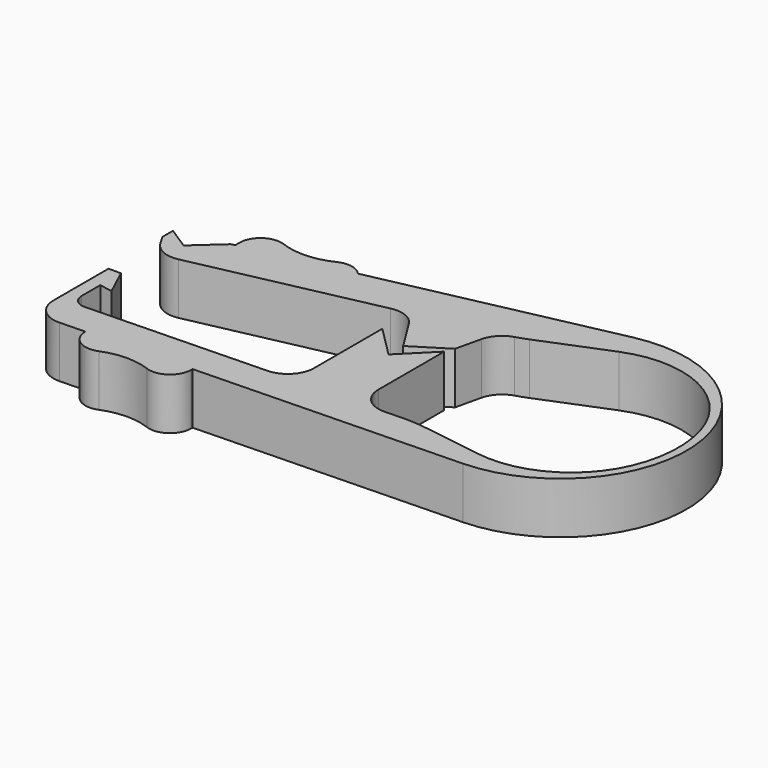
from build123d import *

# Parameters (mm, degrees)
F1_DEPTH     = 5
F2_R         = 12.7
F3_T1_DEPTH  = 5
F3_T3_DEPTH  = 5
F3_T5_DEPTH  = 5
F3_T7_DEPTH  = 5
F3_T9_DEPTH  = 14.2270901057
F3_T11_DEPTH = 18.0454684025
F4_R         = 1.27
F5_R         = 9.652
F6_T1_DEPTH  = 24.5237287856
F6_T3_DEPTH  = 20.8349691576
F6_T5_DEPTH  = 25.4326352389


# Not quite as in the source:
# - a fillet or chamfer that OpenCascade refuses, or shapes differently, is made with other operations: its cross-section is extruded or revolved along the edge and cut away or added


with BuildPart() as f1:
    # F0 (on Top) → F1 (new body)
    with BuildSketch(Plane.XY):
        Polygon((3.3509032068, 2.0938767152), (4.2717468935, 6.0824889279), (5.2645709983, 10.3828825854), (-0.7663700033, 9.1009665025), (-1.7591941081, 4.800572845), (-2.0938767152, 3.3509032068), (0, 0), align=None)
        with BuildLine():
            ThreePointArc((19.0271173058, -10.7843702882), (13.5579507926, -11.3055566189), (8.4773948837, -9.2147746604))
            Line((8.4773948837, -9.2147746604), (3, -9.3617991862))
            Line((3, -9.3617991862), (-3, -9.5228515064))
            Line((-3, -9.5228515064), (-24.13, -10.0900240941))
            Line((-24.13, -10.0900240941), (-24.13, -6.5340240941))
            Line((-24.13, -6.5340240941), (-24.13, -4.0344355705))
            Line((-24.13, -4.0344355705), (-25.33, -4.0344355705))
            Line((-25.33, -4.0344355705), (-25.33, -13.3233871439))
            Line((-25.33, -13.3233871439), (-20.25, -13.1870295128))
            Line((-20.25, -13.1870295128), (-10.09, -12.9143142505))
            Line((-10.09, -12.9143142505), (15.568160115, -12.2255965474))
            ThreePointArc((15.568160115, -12.2255965474), (27.3847553183, 1.4414639293), (12.6972400213, 11.962745157))
            Line((12.6972400213, 11.962745157), (5.2645709983, 10.3828825854))
            Line((5.2645709983, 10.3828825854), (4.2717468935, 6.0824889279))
            Line((4.2717468935, 6.0824889279), (5.7705051289, 6.4010598252))
            ThreePointArc((5.7705051289, 6.4010598252), (10.9582466373, 10.5977114577), (17.6052347625, 11.1826009729))
            ThreePointArc((17.6052347625, 11.1826009729), (26.6461306142, 0.7382983213), (19.0271173058, -10.7843702882))
        make_face()
        Polygon((-24.13, -4.0344355705), (-24.13, -6.5340240941), (-22.86, -6.7579593596), align=None)
        Polygon((-3, -9.5228515064), (3, -9.3617991862), (3, 1.222), (0, -1.778), (-3, 1.222), align=None)
        Polygon((-1.7591941081, 4.800572845), (-0.7663700033, 9.1009665025), (-10.09, 7.1191677681), (-20.25, 4.9595931015), (-20.6003244103, 4.8851293494), (-23.2697767574, 2.48154366), (-25.4, 3.8649268089), (-25.4, 2.5949268089), (-23.9501636865, 0.0837366513), align=None)
        with BuildLine():
            Line((5.7705051289, 6.4010598252), (17.6052347625, 11.1826009729))
            ThreePointArc((17.6052347625, 11.1826009729), (10.9582466373, 10.5977114577), (5.7705051289, 6.4010598252))
        make_face()
        with BuildLine():
            Line((19.0271173058, -10.7843702882), (8.4773948837, -9.2147746604))
            ThreePointArc((8.4773948837, -9.2147746604), (13.5579507926, -11.3055566189), (19.0271173058, -10.7843702882))
        make_face()
        with BuildLine():
            Line((-20.25, 4.9595931015), (-10.09, 7.1191677681))
            Line((-10.09, 7.1191677681), (-10.09, 9.660082633))
            ThreePointArc((-10.09, 9.660082633), (-15.1017802383, 6.9821995552), (-20.25, 9.3873673708))
            Line((-20.25, 9.3873673708), (-20.25, 4.9595931015))
        make_face()
        with BuildLine():
            Line((-10.09, -17.0008412983), (-10.09, -12.9143142505))
            Line((-10.09, -12.9143142505), (-20.25, -13.1870295128))
            Line((-20.25, -13.1870295128), (-20.25, -17.2735565605))
            ThreePointArc((-20.25, -17.2735565605), (-15.2382197617, -14.5956734827), (-10.09, -17.0008412983))
        make_face()
    extrude(amount=F1_DEPTH)

    # F2
    f2_edges = [f1.edges().sort_by_distance(p)[0] for p in [
        (5.770505, 6.40106, 2.5),
        (8.477395, -9.214775, 2.5),
    ]]
    fillet(f2_edges, radius=F2_R)

    # F3: fillet of radius 2.54 on 8 edges, made by hand

    # F3_s2 → F3_t1 (join)
    with BuildSketch(Plane.XY):
        with BuildLine():
            ThreePointArc((5.6695141413, 6.421250807), (4.5433342643, 5.7258928643), (3.9198768127, 4.5583721621))
            Line((3.9198768127, 4.5583721621), (3.6723868163, 4.6155097299))
            Line((3.6723868163, 4.6155097299), (4.024256897, 6.1396264957))
            Line((4.024256897, 6.1396264957), (4.218937324, 6.3309384185))
            ThreePointArc((4.218937324, 6.3309384185), (4.6308698651, 6.4184973831), (5.5969878777, 6.6646762393))
            Line((5.5969878777, 6.6646762393), (5.6695141413, 6.421250807))
        make_face()
    extrude(amount=F3_T1_DEPTH)

    # F3_s4 → F3_t3 (join)
    with BuildSketch(Plane.XY):
        with BuildLine():
            ThreePointArc((-2.0938767152, 3.3509032068), (-3.2128527644, 4.1204303422), (-4.5683542412, 4.2034674259))
            Line((-4.5683542412, 4.2034674259), (-1.7591941081, 4.800572845))
            Line((-1.7591941081, 4.800572845), (-2.0938767152, 3.3509032068))
        make_face()
    extrude(amount=F3_T3_DEPTH)

    # F3_s6 → F3_t5 (join)
    with BuildSketch(Plane.XY):
        with BuildLine():
            ThreePointArc((5.6081542675, -9.2917909701), (3.7682087933, -8.5726933957), (3, -6.7527055057))
            Line((3, -6.7527055057), (3, -9.3617991862))
            Line((3, -9.3617991862), (5.6081542675, -9.2917909701))
        make_face()
    extrude(amount=F3_T5_DEPTH)

    # F3_s8 → F3_t7 (join)
    with BuildSketch(Plane.XY):
        with BuildLine():
            ThreePointArc((-3, -7.050115457), (-3.72001211, -8.8219066637), (-5.4718457325, -9.5892009215))
            Line((-5.4718457325, -9.5892009215), (-3, -9.5228515064))
            Line((-3, -9.5228515064), (-3, -7.050115457))
        make_face()
    extrude(amount=F3_T7_DEPTH)

    # F3_s10 → F3_t9 (cut)
    with BuildSketch(Plane.XY.offset(-4.6135450528)):
        with BuildLine():
            ThreePointArc((-24.872872697, 1.6819155382), (-23.7062792448, 0.6315100757), (-22.1450724768, 0.4674206323))
            Line((-22.1450724768, 0.4674206323), (-23.9501636865, 0.0837366513))
            Line((-23.9501636865, 0.0837366513), (-24.872872697, 1.6819155382))
        make_face()
    extrude(amount=F3_T9_DEPTH, mode=Mode.SUBTRACT)

    # F3_s12 → F3_t11 (cut)
    with BuildSketch(Plane.XY.offset(-6.5227342013)):
        with BuildLine():
            ThreePointArc((-22.7218457325, -13.2533789278), (-24.5617912067, -12.5342813534), (-25.33, -10.7142934634))
            Line((-25.33, -10.7142934634), (-25.33, -13.3233871439))
            Line((-25.33, -13.3233871439), (-22.7218457325, -13.2533789278))
        make_face()
    extrude(amount=F3_T11_DEPTH, mode=Mode.SUBTRACT)

    # F4
    f4_edges = [f1.edges().sort_by_distance(p)[0] for p in [
        (-24.13, -10.090024, 2.5),
    ]]
    fillet(f4_edges, radius=F4_R)

    # F5
    f5_edges = [f1.edges().sort_by_distance(p)[0] for p in [
        (17.605235, 11.182601, 2.5),
        (19.027117, -10.78437, 2.5),
    ]]
    fillet(f5_edges, radius=F5_R)

    # F6: fillet of radius 2.032 on 4 edges, made by hand

    # F6_s2 → F6_t1 (cut)
    with BuildSketch(Plane.XY.offset(-9.7618643928)):
        with BuildLine():
            ThreePointArc((-20.25, 5.4826216137), (-19.3751275367, 7.152974829), (-17.5038584017, 7.3849953356))
            ThreePointArc((-17.5038584017, 7.3849953356), (-19.0133811971, 8.1990450487), (-20.25, 9.3873673708))
            Line((-20.25, 9.3873673708), (-20.25, 5.4826216137))
        make_face()
        with BuildLine():
            ThreePointArc((-12.8361415983, -14.9984692631), (-10.9648724633, -14.7664487565), (-10.09, -13.0960955412))
            Line((-10.09, -13.0960955412), (-10.09, -17.0008412983))
            ThreePointArc((-10.09, -17.0008412983), (-11.3266188029, -15.8125189761), (-12.8361415983, -14.9984692631))
        make_face()
    extrude(amount=F6_T1_DEPTH, mode=Mode.SUBTRACT)

    # F6_s4 → F6_t3 (cut)
    with BuildSketch(Plane.XY.offset(-7.9174845788)):
        with BuildLine():
            ThreePointArc((-12.5069745437, 7.613601755), (-11.2148663887, 7.7751542861), (-10.09, 7.1191677681))
            Line((-10.09, 7.1191677681), (-10.09, 9.660082633))
            ThreePointArc((-10.09, 9.660082633), (-11.1688571334, 8.4837438934), (-12.5069745437, 7.613601755))
        make_face()
    extrude(amount=F6_T3_DEPTH, mode=Mode.SUBTRACT)

    # F6_s6 → F6_t5 (cut)
    with BuildSketch(Plane.XY.offset(-10.2163176194)):
        with BuildLine():
            ThreePointArc((-20.25, -13.1870295128), (-19.3485712422, -14.8643401762), (-17.4543465947, -15.0589111198))
            ThreePointArc((-17.4543465947, -15.0589111198), (-19.0108515696, -15.9659266289), (-20.25, -17.2735565605))
            Line((-20.25, -17.2735565605), (-20.25, -13.1870295128))
        make_face()
    extrude(amount=F6_T5_DEPTH, mode=Mode.SUBTRACT)


solid = f1.part
